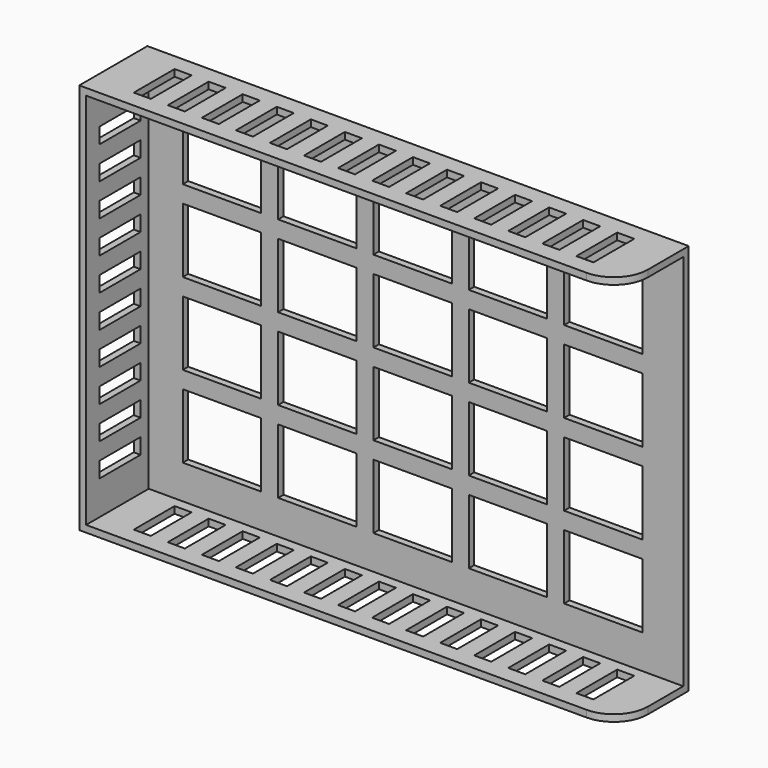
from build123d import *

# Parameters (mm, degrees)
F0_W     = 159
F0_H     = 115
F1_DEPTH = 25
F2_T     = -2
F3_R     = 10
F4_W     = 23
F4_H     = 19
F5_DEPTH = 25
F6_W     = 5
F6_H     = 15
F7_DEPTH = 115.001
F8_W     = 15
F8_H     = 4.6
F9_DEPTH = 25


with BuildPart() as f1:
    # F0 (on Front) → F1 (new body)
    with BuildSketch(Plane.XZ):
        with Locations((-32.5192203745, 11.7968884611)):
            Rectangle(F0_W, F0_H)
    extrude(amount=F1_DEPTH)

    # F2
    f2_openings = [f1.faces().sort_by_distance(p)[0] for p in [
        (-32.51922, -25, 11.796888),
        (46.98078, -12.5, 11.796888),
    ]]
    offset(amount=F2_T, openings=f2_openings)

    # F3
    f3_edges = [f1.edges().sort_by_distance(p)[0] for p in [
        (46.98078, -25, -44.703112),
        (46.98078, -25, 68.296888),
    ]]
    fillet(f3_edges, radius=F3_R)

    # F4 (on face) → F5 (cut)
    with BuildSketch(Plane.XZ.offset(2)):
        with Locations((-88.5192203745, 47.7968884611)):
            Rectangle(F4_W, F4_H)
        with Locations((-60.5192203745, 47.7968884611)):
            Rectangle(F4_W, F4_H)
        with Locations((-32.5192203745, 47.7968884611)):
            Rectangle(F4_W, F4_H)
        with Locations((-4.5192203745, 47.7968884611)):
            Rectangle(F4_W, F4_H)
        with Locations((23.4807796255, 47.7968884611)):
            Rectangle(F4_W, F4_H)
        with Locations((-88.5192203745, 23.7968884611)):
            Rectangle(F4_W, F4_H)
        with Locations((-60.5192203745, 23.7968884611)):
            Rectangle(F4_W, F4_H)
        with Locations((-32.5192203745, 23.7968884611)):
            Rectangle(F4_W, F4_H)
        with Locations((-4.5192203745, 23.7968884611)):
            Rectangle(F4_W, F4_H)
        with Locations((23.4807796255, 23.7968884611)):
            Rectangle(F4_W, F4_H)
        with Locations((23.4807796255, -0.2031115389)):
            Rectangle(F4_W, F4_H)
        with Locations((-4.5192203745, -0.2031115389)):
            Rectangle(F4_W, F4_H)
        with Locations((-32.5192203745, -0.2031115389)):
            Rectangle(F4_W, F4_H)
        with Locations((-60.5192203745, -0.2031115389)):
            Rectangle(F4_W, F4_H)
        with Locations((-88.5192203745, -0.2031115389)):
            Rectangle(F4_W, F4_H)
        with Locations((-88.5192203745, -24.2031115389)):
            Rectangle(F4_W, F4_H)
        with Locations((-60.5192203745, -24.2031115389)):
            Rectangle(F4_W, F4_H)
        with Locations((-32.5192203745, -24.2031115389)):
            Rectangle(F4_W, F4_H)
        with Locations((-4.5192203745, -24.2031115389)):
            Rectangle(F4_W, F4_H)
        with Locations((23.4807796255, -24.2031115389)):
            Rectangle(F4_W, F4_H)
    extrude(amount=-F5_DEPTH, mode=Mode.SUBTRACT)

    # F6 (on face) → F7 (cut, through all)
    with BuildSketch(Plane(origin=(0, 0, -45.7031115389), x_dir=(1, 0, 0), z_dir=(0, 0, -1))):
        with Locations((-97.5192203745, 12.5)):
            Rectangle(F6_W, F6_H)
        with Locations((-87.5192203745, 12.5)):
            Rectangle(F6_W, F6_H)
        with Locations((-77.5192203745, 12.5)):
            Rectangle(F6_W, F6_H)
        with Locations((-67.5192203745, 12.5)):
            Rectangle(F6_W, F6_H)
        with Locations((-57.5192203745, 12.5)):
            Rectangle(F6_W, F6_H)
        with Locations((-47.5192203745, 12.5)):
            Rectangle(F6_W, F6_H)
        with Locations((-37.5192203745, 12.5)):
            Rectangle(F6_W, F6_H)
        with Locations((-27.5192203745, 12.5)):
            Rectangle(F6_W, F6_H)
        with Locations((-17.5192203745, 12.5)):
            Rectangle(F6_W, F6_H)
        with Locations((-7.5192203745, 12.5)):
            Rectangle(F6_W, F6_H)
        with Locations((2.4807796255, 12.5)):
            Rectangle(F6_W, F6_H)
        with Locations((12.4807796255, 12.5)):
            Rectangle(F6_W, F6_H)
        with Locations((22.4807796255, 12.5)):
            Rectangle(F6_W, F6_H)
        with Locations((32.4807796255, 12.5)):
            Rectangle(F6_W, F6_H)
    extrude(amount=-F7_DEPTH, mode=Mode.SUBTRACT)

    # F8 (on face) → F9 (cut)
    with BuildSketch(Plane(origin=(-112.0192203745, 0, 0), x_dir=(0, -1, 0), z_dir=(-1, 0, 0))):
        with Locations((12.5, 54.9968907654)):
            Rectangle(F8_W, F8_H)
        with Locations((12.5, 45.3968907654)):
            Rectangle(F8_W, F8_H)
        with Locations((12.5, 35.7968907654)):
            Rectangle(F8_W, F8_H)
        with Locations((12.5, 26.1968907654)):
            Rectangle(F8_W, F8_H)
        with Locations((12.5, 16.5968907654)):
            Rectangle(F8_W, F8_H)
        with Locations((12.5, 6.9968907654)):
            Rectangle(F8_W, F8_H)
        with Locations((12.5, -2.6031092346)):
            Rectangle(F8_W, F8_H)
        with Locations((12.5, -12.2031092346)):
            Rectangle(F8_W, F8_H)
        with Locations((12.5, -21.8031092346)):
            Rectangle(F8_W, F8_H)
        with Locations((12.5, -31.4031092346)):
            Rectangle(F8_W, F8_H)
    extrude(amount=-F9_DEPTH, mode=Mode.SUBTRACT)


solid = f1.part
